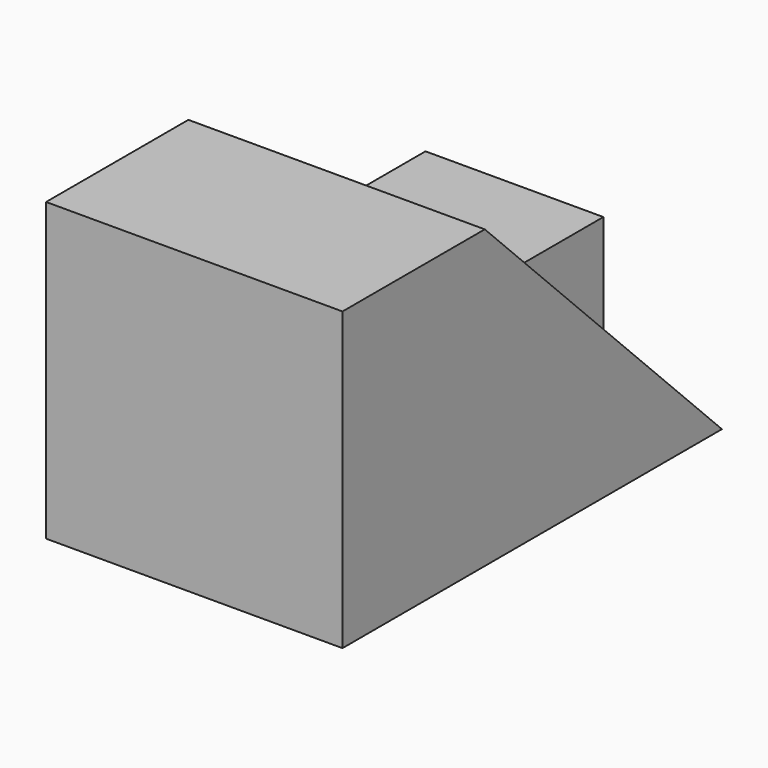
from build123d import *

# Parameters (mm, degrees)
F0_W     = 50.8
F0_H     = 31.75
F1_DEPTH = 31.75
F3_DEPTH = 12.7
F5_DEPTH = 50.8
F7_DEPTH = 25.4


# Not quite as in the source:
# - a feature of the source that left no trace in its solid (it failed there, or was rolled back) is left out


with BuildPart() as f1:
    # F0 (on Right) → F1 (new body)
    with BuildSketch(Plane.YZ):
        with Locations((25.4, 15.875)):
            Rectangle(F0_W, F0_H)
    extrude(amount=F1_DEPTH)

    # F2 (on face) → F3 (cut)
    with BuildSketch(Plane.YZ.offset(31.75)):
        Polygon((19.05, 31.75), (50.8, 0), (50.8, 31.75), align=None)
    extrude(amount=-F3_DEPTH, mode=Mode.SUBTRACT)

    # F4 (on face) → F5 (cut)
    with BuildSketch(Plane.YZ.offset(19.05)):
        Polygon((19.05, 31.75), (34.925, 15.875), (38.1, 31.75), align=None)
    extrude(amount=-F5_DEPTH, mode=Mode.SUBTRACT)

    # F6 (on face) → F7 (cut)
    with BuildSketch(Plane.YZ.offset(19.05)):
        Polygon((38.1, 31.75), (34.925, 15.875), (50.8, 15.875), (50.8, 31.2204860245), align=None)
        Polygon((50.8, 31.75), (38.1, 31.75), (50.8, 31.2204860245), align=None)
    extrude(amount=-F7_DEPTH, mode=Mode.SUBTRACT)


solid = f1.part
